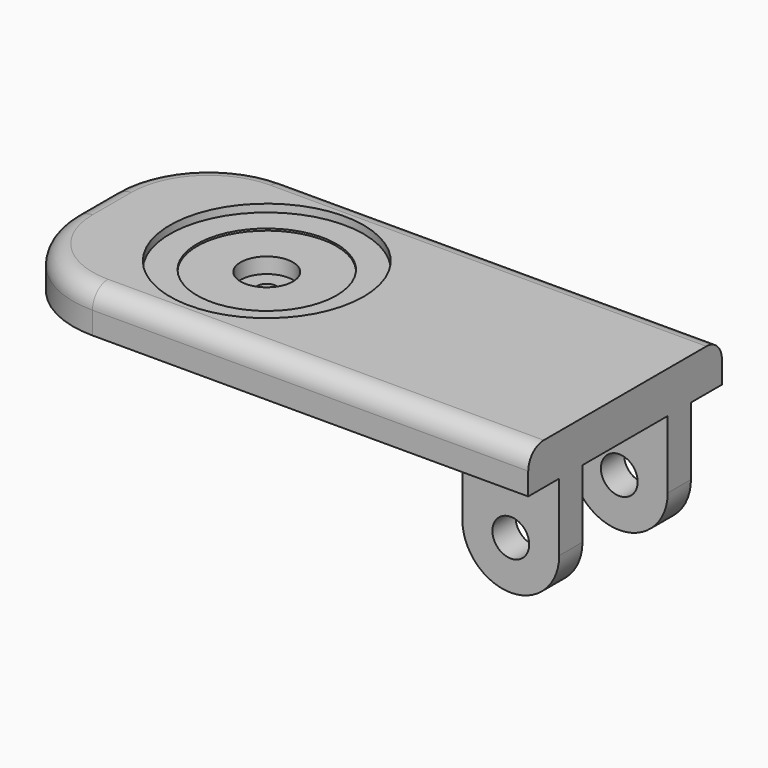
from build123d import *

# Parameters (mm, degrees)
F0_R      = 10
F0_R_2    = 7.2
F0_R_3    = 2.7
F1_DEPTH  = 4.3
F2_DEPTH  = 0.8
F3_DEPTH  = 1
F4_R      = 4.25
F5_DEPTH  = 1
F4_W      = 10
F4_H      = 3
F6_DEPTH  = 12
F8_R      = 4.99999
F7_R      = 1.9
F9_DEPTH  = 25
F10_R     = 2
F11_DEPTH = 2.6
F12_D     = 2


# Not quite as in the source:
# - a fillet or chamfer is up to 0.001 mm smaller than in the source, because OpenCascade refuses the exact size


with BuildPart() as f1:
    # F0 (on Top) → F1 (new body)
    with BuildSketch(Plane.XY):
        with BuildLine():
            Line((0, 12.5), (-45, 12.5))
            ThreePointArc((-45, 12.5), (-52.0710678119, 9.5710678119), (-55, 2.5))
            Line((-55, 2.5), (-55, -2.5))
            ThreePointArc((-55, -2.5), (-52.0710678119, -9.5710678119), (-45, -12.5))
            Line((-45, -12.5), (0, -12.5))
            Line((0, -12.5), (0, 12.5))
        make_face()
        with Locations((-37, 0)):
            Circle(F0_R, mode=Mode.SUBTRACT)
        with Locations((-37, 0)):
            Circle(F0_R)
        with Locations((-37, 0)):
            Circle(F0_R_2, mode=Mode.SUBTRACT)
        with Locations((-37, 0)):
            Circle(F0_R_2)
        with Locations((-37, 0)):
            Circle(F0_R_3, mode=Mode.SUBTRACT)
        with Locations((-37, 0)):
            Circle(F0_R_3)
    extrude(amount=-F1_DEPTH)

    # F0 (on Top) → F2 (cut)
    with BuildSketch(Plane.XY):
        with Locations((-37, 0)):
            Circle(F0_R)
        with Locations((-37, 0)):
            Circle(F0_R_2, mode=Mode.SUBTRACT)
        with Locations((-37, 0)):
            Circle(F0_R_2)
        with Locations((-37, 0)):
            Circle(F0_R_3, mode=Mode.SUBTRACT)
    extrude(amount=-F2_DEPTH, mode=Mode.SUBTRACT)

    # F0 (on Top) → F3 (cut)
    with BuildSketch(Plane.XY):
        with Locations((-37, 0)):
            Circle(F0_R_2)
        with Locations((-37, 0)):
            Circle(F0_R_3, mode=Mode.SUBTRACT)
    extrude(amount=-F3_DEPTH, mode=Mode.SUBTRACT)

    # F4 (on face) → F5 (cut)
    with BuildSketch(Plane(origin=(0, 0, -4.3), x_dir=(1, 0, 0), z_dir=(0, 0, -1))):
        with Locations((-37, 0)):
            Circle(F4_R)
    extrude(amount=-F5_DEPTH, mode=Mode.SUBTRACT)

    # F4 (on face) → F6 (join)
    with BuildSketch(Plane(origin=(0, 0, -4.3), x_dir=(1, 0, 0), z_dir=(0, 0, -1))):
        with Locations((-5, 7)):
            Rectangle(F4_W, F4_H)
        with Locations((-5, -7)):
            Rectangle(F4_W, F4_H)
    extrude(amount=F6_DEPTH)

    # F8 (radius 5 in the source; OpenCascade refuses exactly that, so slightly less here)
    f8_edges = [f1.edges().sort_by_distance(p)[0] for p in [
        (0, -7, -16.3),
        (0, 7, -16.3),
        (-10, 7, -16.3),
        (-10, -7, -16.3),
    ]]
    fillet(f8_edges, radius=F8_R)

    # F7 (on face) → F9 (cut)
    with BuildSketch(Plane.XZ.offset(8.5)):
        with Locations((-5, -11.3)):
            Circle(F7_R)
    extrude(amount=-F9_DEPTH, mode=Mode.SUBTRACT)

    # F10
    f10_edges = [f1.edges().sort_by_distance(p)[0] for p in [
        (-22.5, -12.5, 0),
    ]]
    fillet(f10_edges, radius=F10_R)

    # F11 (cut): a face of the model
    f11_faces = [f1.faces().sort_by_distance(p)[0] for p in [
        (-37, 0, 0),
    ]]
    extrude(f11_faces, amount=-F11_DEPTH, mode=Mode.SUBTRACT)

    # F12 (through all)
    with Locations(Plane.XY):
        with Locations((-37, 0)):
            Hole(F12_D / 2)


solid = f1.part
